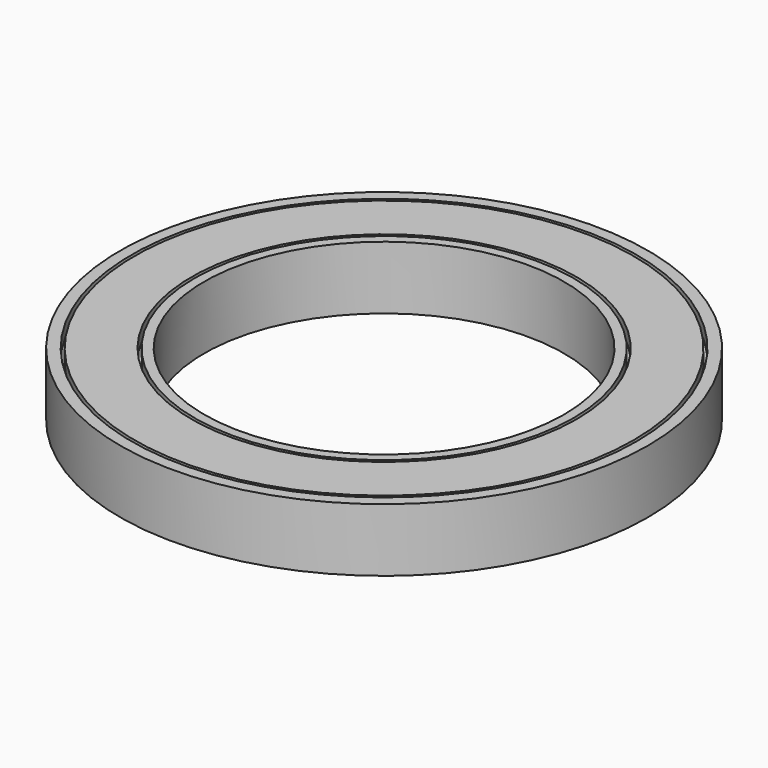
from build123d import *

# Parameters (mm, degrees)
F0_R     = 20.9
F1_DEPTH = 5
F2_R     = 14.25
F3_DEPTH = 25
F4_R     = 20
F4_R_2   = 15
F5_DEPTH = 1
F6_R     = 19.75
F6_R_2   = 15.25
F7_DEPTH = 1
F8_R     = 29.8872921221
F8_R_2   = 20.9
F9_DEPTH = 2.5


# Not quite as in the source:
# - a feature of the source that left no trace in its solid (it failed there, or was rolled back) is left out
# - a pattern or mirror of a feature is missing from the dataset's text; its kind, count and spacing are read off the source's solid


with BuildPart() as f1:
    # F0 (on Top) → F1 (new body)
    with BuildSketch(Plane.XY):
        Circle(F0_R)
    extrude(amount=F1_DEPTH)

    # F2 (on face) → F3 (cut)
    with BuildSketch(Plane.XY.offset(5)):
        Circle(F2_R)
    extrude(amount=-F3_DEPTH, mode=Mode.SUBTRACT)

    # F4 (on face) → F5 (cut)
    with BuildSketch(Plane.XY.offset(5)):
        Circle(F4_R)
        Circle(F4_R_2, mode=Mode.SUBTRACT)
    f5 = extrude(amount=-F5_DEPTH, mode=Mode.SUBTRACT)

    # F5_copies: F5 across plane
    add(f5.mirror(Plane(origin=(0, 0, 2.5), x_dir=(-1, 0, 0), z_dir=(0, 0, -1))), mode=Mode.SUBTRACT)

    # F8 (on face) → F9 (cut)
    with BuildSketch(Plane(origin=(0, 0, 0), x_dir=(1, 0, 0), z_dir=(0, 0, -1))):
        Circle(F8_R)
        Circle(F8_R_2, mode=Mode.SUBTRACT)
    extrude(amount=-F9_DEPTH, mode=Mode.SUBTRACT)


with BuildPart() as f7:
    # F6 (on face) → F7 (new body)
    with BuildSketch(Plane.XY.offset(4)):
        Circle(F6_R)
        Circle(F6_R_2, mode=Mode.SUBTRACT)
    extrude(amount=F7_DEPTH)


with BuildPart() as f7_copies_1:
    # F7_copies: instance of F7
    add(f7.part.mirror(Plane(origin=(0, 0, 2.5), x_dir=(-1, 0, 0), z_dir=(0, 0, -1))))


solid = Compound([f1.part, f7.part, f7_copies_1.part])
